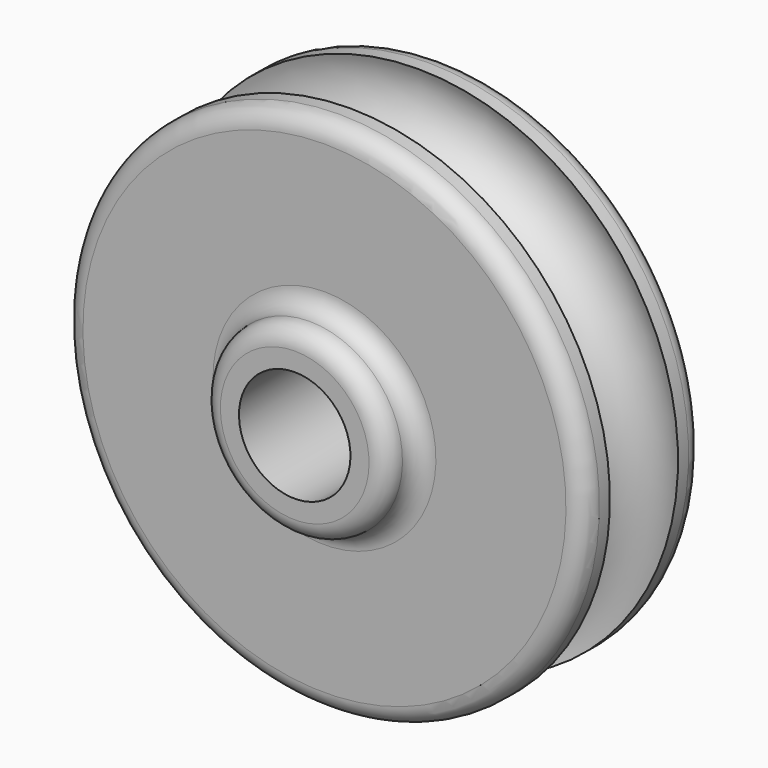
from build123d import *

# Parameters (mm, degrees)
F2_R = 12.69999


# Not quite as in the source:
# - a fillet or chamfer is up to 0.001 mm smaller than in the source, because OpenCascade refuses the exact size


with BuildPart() as f1:
    # F0 (on Right) → F1 (revolve)
    with BuildSketch(Plane.YZ):
        with BuildLine():
            Line((-50.8, 63.5), (50.8, 63.5))
            Line((50.8, 63.5), (50.8, 177.8))
            Line((50.8, 177.8), (29.099355663, 177.8))
            ThreePointArc((29.099355663, 177.8), (0, 133.35), (-29.099355663, 177.8))
            Line((-29.099355663, 177.8), (-50.8, 177.8))
            Line((-50.8, 177.8), (-50.8, 63.5))
        make_face()
        Polygon((76.2, 38.1), (76.2, 63.5), (50.8, 63.5), (-50.8, 63.5), (-76.2, 63.5), (-76.2, 38.1), align=None)
    revolve(axis=Axis((0, 0, 0), (0, 1, 0)))

    # F2 (radius 12.7 in the source; OpenCascade refuses exactly that, so slightly less here)
    f2_edges = [f1.edges().sort_by_distance(p)[0] for p in [
        (0, -50.8, -177.8),
        (0, 50.8, -177.8),
        (0, -76.2, -63.5),
        (0, 76.2, -63.5),
        (0, -50.8, -63.5),
        (0, 50.8, -63.5),
    ]]
    fillet(f2_edges, radius=F2_R)


solid = f1.part
